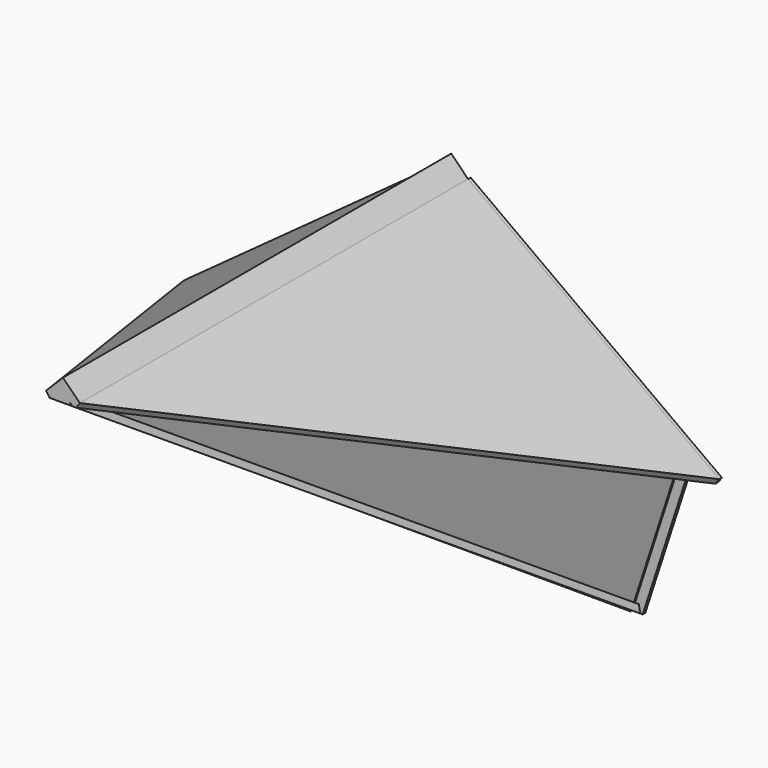
from build123d import *

# Parameters (mm, degrees)
F1_DEPTH  = 50.8
F2_DEPTH  = 7620
F4_DEPTH  = 5016.876130589
F6_DEPTH  = 5016.876130589
F7_DEPTH  = 50.8
F8_DEPTH  = 50.8
F9_DEPTH  = 50.8
F10_DEPTH = 50.8
F13_DEPTH = 101.6
F16_DEPTH = 101.6
F19_DEPTH = 101.6
F20_DEPTH = 7620


# Not quite as in the source:
# - a feature names something its author has since deleted; it is built from what else it names


with BuildPart() as f1:
    # F0 (on Front) → F1 (new body)
    with BuildSketch(Plane.XZ):
        Polygon((3781.2287860666, -1063.8068812603), (-164.1852921012, -3930.3179996402), (-104.4663104683, -4012.5141262687), (224.3181960457, -3773.6381997371), (353.9573792386, -3679.4498198516), (563.7179839184, -3527.0498198516), (3840.9477676995, -1146.0030078888), align=None)
    extrude(amount=-F1_DEPTH)


with BuildPart() as f1b:
    # F0 (on Front) → F1, piece 2 (new body)
    with BuildSketch(Plane.XZ):
        Polygon((8257.8992157481, -3930.3179996402), (4312.4851375803, -1063.8068812603), (4252.7661559474, -1146.0030078888), (7529.9959397285, -3527.0498198516), (7739.7565444083, -3679.4498198516), (7869.3957276012, -3773.6381997371), (8198.1802341152, -4012.5141262687), align=None)
    extrude(amount=-F1_DEPTH)


with BuildPart() as f2:
    # F0 (on Front) → F2 (new body)
    with BuildSketch(Plane.XZ):
        Polygon((8257.8992157481, -3930.3179996402), (4312.4851375803, -1063.8068812603), (4252.7661559474, -1146.0030078888), (7529.9959397285, -3527.0498198516), (7739.7565444083, -3679.4498198516), (7869.3957276012, -3773.6381997371), (8198.1802341152, -4012.5141262687), align=None)
    extrude(amount=F2_DEPTH)

    # F3 (on face) → F4 (cut, through all)
    with BuildSketch(Plane(origin=(984.0567377882, 0, 1354.4379026095), x_dir=(0.8090169944, 0, -0.5877852523), z_dir=(0.5877852523, 0, 0.8090169944))):
        Polygon((8990.9637603839, 0), (4114.1637603839, -7620), (8990.9637603839, -7620), align=None)
    extrude(amount=-F4_DEPTH, mode=Mode.SUBTRACT)


with BuildPart() as f2b:
    # F0 (on Front) → F2, piece 2 (new body)
    with BuildSketch(Plane.XZ):
        Polygon((3781.2287860666, -1063.8068812603), (-164.1852921012, -3930.3179996402), (-104.4663104683, -4012.5141262687), (224.3181960457, -3773.6381997371), (353.9573792386, -3679.4498198516), (563.7179839184, -3527.0498198516), (3840.9477676995, -1146.0030078888), align=None)
    extrude(amount=F2_DEPTH)

    # F5 (on face) → F6 (cut, through all)
    with BuildSketch(Plane(origin=(1812.2526490272, 0, -2494.3517814471), x_dir=(0.8090169944, 0, 0.5877852523), z_dir=(-0.5877852523, 0, 0.8090169944))):
        Polygon((-2443.0116485444, -7620), (2433.7883514556, -7620), (-2443.0116485444, 0), align=None)
    extrude(amount=-F6_DEPTH, mode=Mode.SUBTRACT)


with BuildPart() as f7:
    # F0 (on Front) → F7 (new body)
    with BuildSketch(Plane.XZ):
        Polygon((4252.7661559474, -1146.0030078888), (4046.8569618235, -1146.0030078888), (5363.4444852873, -3527.0498198516), (5569.3536794113, -3527.0498198516), align=None)
    extrude(amount=F7_DEPTH)


with BuildPart() as f7b:
    # F0 (on Front) → F7, piece 2 (new body)
    with BuildSketch(Plane.XZ):
        Polygon((4046.8569618235, -1146.0030078888), (3840.9477676995, -1146.0030078888), (2524.3602442356, -3527.0498198516), (2730.2694383596, -3527.0498198516), align=None)
    extrude(amount=F7_DEPTH)


with BuildPart() as f8:
    # F0 (on Front) → F8 (new body)
    with BuildSketch(Plane.XZ):
        Polygon((353.9573792386, -3679.4498198516), (224.3181960457, -3773.6381997371), (998.8569618235, -6157.4234080753), (7094.8569618235, -6157.4234080753), (7869.3957276012, -3773.6381997371), (7739.7565444083, -3679.4498198516), (6967.6259599868, -6055.8234080753), (6761.7167658628, -6055.8234080753), (1331.9971577841, -6055.8234080753), (1126.0879636601, -6055.8234080753), align=None)
    extrude(amount=F8_DEPTH)


with BuildPart() as f9:
    # F0 (on Front) → F9 (new body)
    with BuildSketch(Plane.XZ):
        Polygon((5653.6224714266, -3679.4498198516), (5447.7132773026, -3679.4498198516), (6761.7167658628, -6055.8234080753), (6967.6259599868, -6055.8234080753), align=None)
    extrude(amount=F9_DEPTH)


with BuildPart() as f9b:
    # F0 (on Front) → F9, piece 2 (new body)
    with BuildSketch(Plane.XZ):
        Polygon((7739.7565444083, -3679.4498198516), (7529.9959397285, -3527.0498198516), (5569.3536794113, -3527.0498198516), (5653.6224714266, -3679.4498198516), align=None)
    extrude(amount=F9_DEPTH)


with BuildPart() as f9c:
    # F0 (on Front) → F9, piece 3 (new body)
    with BuildSketch(Plane.XZ):
        Polygon((2524.3602442356, -3527.0498198516), (563.7179839184, -3527.0498198516), (353.9573792386, -3679.4498198516), (2440.0914522204, -3679.4498198516), align=None)
    extrude(amount=F9_DEPTH)


with BuildPart() as f9d:
    # F0 (on Front) → F9, piece 4 (new body)
    with BuildSketch(Plane.XZ):
        Polygon((2646.0006463443, -3679.4498198516), (2440.0914522204, -3679.4498198516), (1126.0879636601, -6055.8234080753), (1331.9971577841, -6055.8234080753), align=None)
    extrude(amount=F9_DEPTH)


with BuildPart() as f10:
    # F0 (on Front) → F10 (new body)
    with BuildSketch(Plane.XZ):
        Polygon((5363.4444852873, -3527.0498198516), (2730.2694383596, -3527.0498198516), (2646.0006463443, -3679.4498198516), (5447.7132773026, -3679.4498198516), align=None)
    extrude(amount=F10_DEPTH)


with BuildPart() as f13:
    # F12 (on 3pt) → F13 (new body)
    with BuildSketch(Plane(origin=(0, -2849.7769817203, -4304.2750772285), x_dir=(1, 0, 0), z_dir=(0, 0.5520500585, 0.8338109695))):
        Polygon((4239.7484779358, -5703.8235664368), (7065.0205612183, 3387.3665332794), (962.1124267578, 3387.3665332794), (3817.0967102051, -5703.8235664368), align=None)
    extrude(amount=F13_DEPTH)


with BuildPart() as f16:
    # F15 (on face) → F16 (new body)
    with BuildSketch(Plane(origin=(6219.7211580064, -3656.1622452923, -2020.9099093128), x_dir=(0.4640972567, 0.8728543999, -0.1507943397), z_dir=(0.8301338648, -0.4879807338, -0.2697268432))):
        Polygon((4054.3885231018, -1155.7741165161), (-4555.5882453918, 228.5533994436), (4054.3885231018, -3681.804895401), align=None)
    extrude(amount=-F16_DEPTH)


with BuildPart() as f19:
    # F18 (on face) → F19 (new body)
    with BuildSketch(Plane(origin=(-727.4852094478, -430.4918680103, -236.3742732677), x_dir=(-0.4664493221, 0.8714671704, -0.151558572), z_dir=(0.8288145312, 0.4904538417, 0.2692981657))):
        Polygon((-8228.2686233521, -2277.9448032379), (436.1208975315, -6154.6440124512), (415.3425097466, -3674.2062568665), align=None)
    extrude(amount=F19_DEPTH)


with BuildPart() as f20:
    # F0 (on Front) → F20 (new body)
    with BuildSketch(Plane.XZ):
        Polygon((4046.8569618235, -798.1787055034), (3781.2287860666, -1063.8068812603), (3840.9477676995, -1146.0030078888), (4046.8569618235, -1146.0030078888), (4252.7661559474, -1146.0030078888), (4312.4851375803, -1063.8068812603), align=None)
    extrude(amount=F20_DEPTH)


solid = Compound([f1.part, f1b.part, f2.part, f2b.part, f7.part, f7b.part, f8.part, f9.part, f9b.part, f9c.part, f9d.part, f10.part, f13.part, f16.part, f19.part, f20.part])
